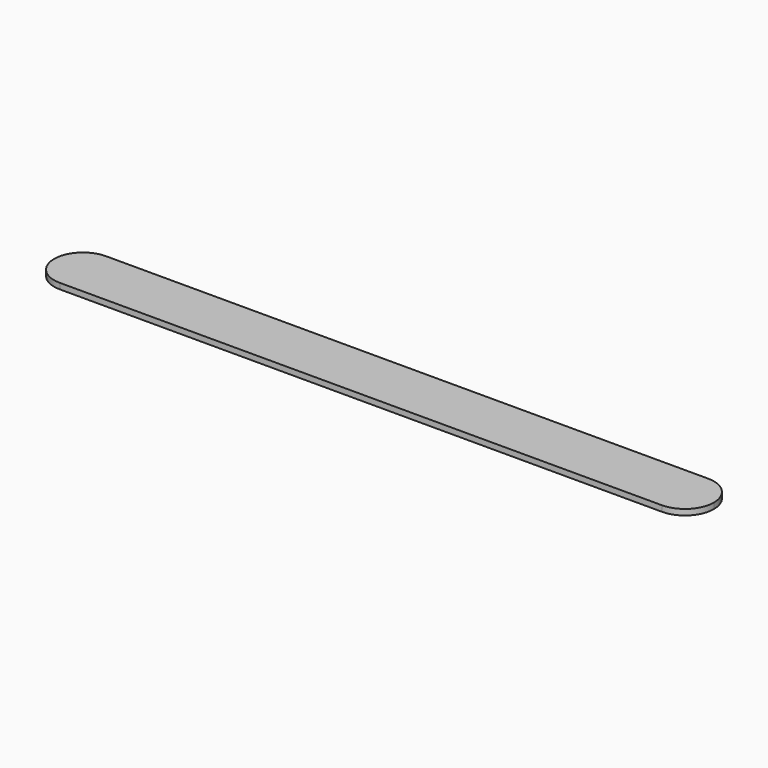
from build123d import *

# Parameters (mm, degrees)
F1_DEPTH = 1


# Not quite as in the source:
# - ends of sketch curves that miss each other by under 0.0002 mm in the source are joined


with BuildPart() as f1:
    # F0 (on Top) → F1 (new body)
    with BuildSketch(Plane.XY):
        with BuildLine():
            Line((60.1628566616, 10), (-44.1295433384, 10))
            ThreePointArc((-44.1295433384, 10), (-47.6650762263, 8.5371068949), (-49.1333375668, 5.0037999912))
            Line((-49.1333375668, 5.0037999912), (-49.1333433384, 4.9962))
            ThreePointArc((-49.1333433384, 4.9962), (-47.6650762263, 1.4628931051), (-44.1295433384, 0))
            Line((-44.1295433384, 0), (60.1628566616, 0))
            ThreePointArc((60.1628566616, 0), (63.6983895496, 1.4628931051), (65.16665089, 4.9962000088))
            Line((65.16665089, 4.9962000088), (65.1666566616, 5.0038))
            ThreePointArc((65.1666566616, 5.0038), (63.6983895496, 8.5371068949), (60.1628566616, 10))
        make_face()
    extrude(amount=F1_DEPTH)


solid = f1.part
